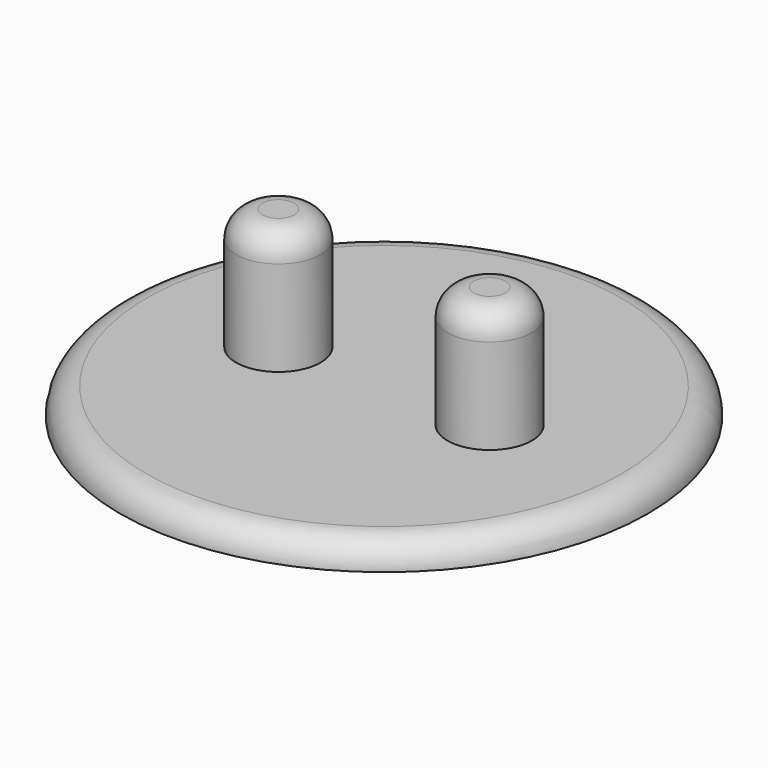
from build123d import *

# Parameters (mm, degrees)
F0_R     = 10
F0_R_2   = 1.6
F1_DEPTH = 1
F2_DEPTH = 4.6
F3_R     = 1
F4_R     = 0.99999


# Not quite as in the source:
# - a fillet or chamfer is up to 0.001 mm smaller than in the source, because OpenCascade refuses the exact size


with BuildPart() as f1:
    # F0 (on Top) → F1 (new body)
    with BuildSketch(Plane.XY):
        Circle(F0_R)
        with Locations((-4, 0)):
            Circle(F0_R_2, mode=Mode.SUBTRACT)
        with Locations((4, 0)):
            Circle(F0_R_2, mode=Mode.SUBTRACT)
        with Locations((-4, 0)):
            Circle(F0_R_2)
        with Locations((4, 0)):
            Circle(F0_R_2)
    extrude(amount=-F1_DEPTH)

    # F0 (on Top) → F2 (join)
    with BuildSketch(Plane.XY):
        with Locations((-4, 0)):
            Circle(F0_R_2)
        with Locations((4, 0)):
            Circle(F0_R_2)
    extrude(amount=F2_DEPTH)

    # F3
    f3_edges = [f1.edges().sort_by_distance(p)[0] for p in [
        (-5.6, 0, 4.6),
        (2.4, 0, 4.6),
    ]]
    fillet(f3_edges, radius=F3_R)

    # F4 (radius 1 in the source; OpenCascade refuses exactly that, so slightly less here)
    f4_edges = [f1.edges().sort_by_distance(p)[0] for p in [
        (-10, 0, 0),
    ]]
    fillet(f4_edges, radius=F4_R)


solid = f1.part
